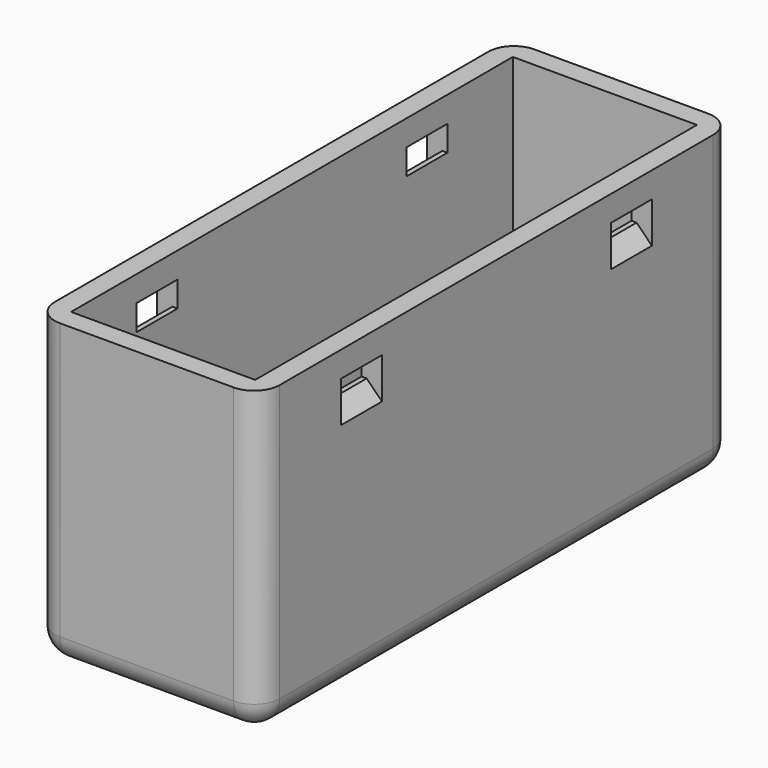
from build123d import *

# Parameters (mm, degrees)
F0_W         = 36
F0_H         = 108
F1_DEPTH     = 55
F2_T         = 4
F3_T1_DEPTH  = 66.5
F3_T3_DEPTH  = 34
F3_T5_DEPTH  = 106
F3_S9_W      = 5
F3_S9_H      = 5
F3_T10_DEPTH = 5
F3_S15_W     = 5
F3_S15_H     = 5
F3_T16_DEPTH = 5
F3_S21_W     = 5
F3_S21_H     = 5
F3_T22_DEPTH = 5
F3_S27_W     = 5
F3_S27_H     = 5
F3_T28_DEPTH = 5
F4_W         = 10
F4_H         = 5
F5_DEPTH     = 44.001
F6_SIZE      = 3


# Not quite as in the source:
# - a fillet or chamfer that OpenCascade refuses, or shapes differently, is made with other operations: its cross-section is extruded or revolved along the edge and cut away or added


with BuildPart() as f1:
    # F0 (on Top) → F1 (new body)
    with BuildSketch(Plane.XY):
        Rectangle(F0_W, F0_H)
    extrude(amount=F1_DEPTH)

    # F2
    f2_openings = [f1.faces().sort_by_distance(p)[0] for p in [
        (0, 0, 55),
    ]]
    offset(amount=F2_T, openings=f2_openings, kind=Kind.INTERSECTION)

    # F3: fillet of radius 5 on 8 edges, made by hand

    # F3_s2 → F3_t1 (cut)
    with BuildSketch(Plane.XY.offset(1)):
        with BuildLine():
            ThreePointArc((-17, -58), (-20.5355339059, -56.5355339059), (-22, -53))
            Line((-22, -53), (-22, -58))
            Line((-22, -58), (-17, -58))
        make_face()
        with BuildLine():
            ThreePointArc((17, -58), (20.5355339059, -56.5355339059), (22, -53))
            Line((22, -53), (22, -58))
            Line((22, -58), (17, -58))
        make_face()
        with BuildLine():
            ThreePointArc((22, 53), (20.5355339059, 56.5355339059), (17, 58))
            Line((17, 58), (22, 58))
            Line((22, 58), (22, 53))
        make_face()
        with BuildLine():
            ThreePointArc((-17, 58), (-20.5355339059, 56.5355339059), (-22, 53))
            Line((-22, 53), (-22, 58))
            Line((-22, 58), (-17, 58))
        make_face()
    extrude(amount=F3_T1_DEPTH, mode=Mode.SUBTRACT)

    # F3_s4 → F3_t3 (cut)
    with BuildSketch(Plane.YZ.offset(-17)):
        with BuildLine():
            ThreePointArc((-58, 1), (-56.5355339059, -2.5355339059), (-53, -4))
            Line((-53, -4), (-58, -4))
            Line((-58, -4), (-58, 1))
        make_face()
        with BuildLine():
            ThreePointArc((58, 1), (56.5355339059, -2.5355339059), (53, -4))
            Line((53, -4), (58, -4))
            Line((58, -4), (58, 1))
        make_face()
    extrude(amount=F3_T3_DEPTH, mode=Mode.SUBTRACT)

    # F3_s6 → F3_t5 (cut)
    with BuildSketch(Plane.XZ.offset(-53)):
        with BuildLine():
            ThreePointArc((22, 1), (20.5355339059, -2.5355339059), (17, -4))
            Line((17, -4), (22, -4))
            Line((22, -4), (22, 1))
        make_face()
        with BuildLine():
            ThreePointArc((-22, 1), (-20.5355339059, -2.5355339059), (-17, -4))
            Line((-17, -4), (-22, -4))
            Line((-22, -4), (-22, 1))
        make_face()
    extrude(amount=F3_T5_DEPTH, mode=Mode.SUBTRACT)


with BuildPart() as f3_tool8:
    # F3_s9 → F3_t10 (new body)
    with BuildSketch(Plane.YZ.offset(-17)):
        with Locations((-55.5, -1.5)):
            Rectangle(F3_S9_W, F3_S9_H)
    extrude(amount=-F3_T10_DEPTH)

    # F3_s11 → F3_t12 (revolve, cut)
    with BuildSketch(Plane(origin=(-17, -53, 1), x_dir=(0, 0.7071067812, 0.7071067812), z_dir=(0, -0.7071067812, 0.7071067812))):
        with BuildLine():
            ThreePointArc((0, -5), (5, 0), (0, 5))
            Line((0, 5), (0, -5))
        make_face()
    revolve(axis=Axis((-17, -53, 1), (-1, 0, 0)), mode=Mode.SUBTRACT)


with BuildPart() as f1_1:
    add(f1.part)

    # F3_t7: cut F3_tool8
    add(f3_tool8.part, mode=Mode.SUBTRACT)


with BuildPart() as f3_tool14:
    # F3_s15 → F3_t16 (new body)
    with BuildSketch(Plane.XY.offset(1)):
        with Locations((19.5, -55.5)):
            Rectangle(F3_S15_W, F3_S15_H)
    extrude(amount=-F3_T16_DEPTH)

    # F3_s17 → F3_t18 (revolve, cut)
    with BuildSketch(Plane(origin=(17, -53, 1), x_dir=(-0.7071067812, 0.7071067812, 0), z_dir=(-0.7071067812, -0.7071067812, 0))):
        with BuildLine():
            ThreePointArc((0, -5), (5, 0), (0, 5))
            Line((0, 5), (0, -5))
        make_face()
    revolve(axis=Axis((17, -53, 1), (0, 0, -1)), mode=Mode.SUBTRACT)


with BuildPart() as f1_2:
    add(f1_1.part)

    # F3_t13: cut F3_tool14
    add(f3_tool14.part, mode=Mode.SUBTRACT)


with BuildPart() as f3_tool20:
    # F3_s21 → F3_t22 (new body)
    with BuildSketch(Plane.XZ.offset(-53)):
        with Locations((19.5, -1.5)):
            Rectangle(F3_S21_W, F3_S21_H)
    extrude(amount=-F3_T22_DEPTH)

    # F3_s23 → F3_t24 (revolve, cut)
    with BuildSketch(Plane(origin=(17, 53, 1), x_dir=(-0.7071067812, 0, 0.7071067812), z_dir=(-0.7071067812, 0, -0.7071067812))):
        with BuildLine():
            ThreePointArc((0, -5), (5, 0), (0, 5))
            Line((0, 5), (0, -5))
        make_face()
    revolve(axis=Axis((17, 53, 1), (0, 1, 0)), mode=Mode.SUBTRACT)


with BuildPart() as f1_3:
    add(f1_2.part)

    # F3_t19: cut F3_tool20
    add(f3_tool20.part, mode=Mode.SUBTRACT)


with BuildPart() as f3_tool26:
    # F3_s27 → F3_t28 (new body)
    with BuildSketch(Plane.XZ.offset(-53)):
        with Locations((-19.5, -1.5)):
            Rectangle(F3_S27_W, F3_S27_H)
    extrude(amount=-F3_T28_DEPTH)

    # F3_s29 → F3_t30 (revolve, cut)
    with BuildSketch(Plane(origin=(-17, 53, 1), x_dir=(0.7071067812, 0, 0.7071067812), z_dir=(-0.7071067812, 0, 0.7071067812))):
        with BuildLine():
            ThreePointArc((0, -5), (5, 0), (0, 5))
            Line((0, 5), (0, -5))
        make_face()
    revolve(axis=Axis((-17, 53, 1), (0, 1, 0)), mode=Mode.SUBTRACT)


with BuildPart() as f1_4:
    add(f1_3.part)

    # F3_t25: cut F3_tool26
    add(f3_tool26.part, mode=Mode.SUBTRACT)

    # F4 (on face) → F5 (cut, through all)
    with BuildSketch(Plane(origin=(-22, 0, 0), x_dir=(0, -1, 0), z_dir=(-1, 0, 0))):
        with Locations((-33, 47.5)):
            Rectangle(F4_W, F4_H)
        with Locations((33, 47.5)):
            Rectangle(F4_W, F4_H)
    extrude(amount=-F5_DEPTH, mode=Mode.SUBTRACT)

    # F6
    f6_edges = [f1_4.edges().sort_by_distance(p)[0] for p in [
        (-22, 33, 45),
        (-22, -33, 45),
        (22, -33, 45),
        (22, 33, 45),
    ]]
    chamfer(f6_edges, length=F6_SIZE)


solid = f1_4.part
